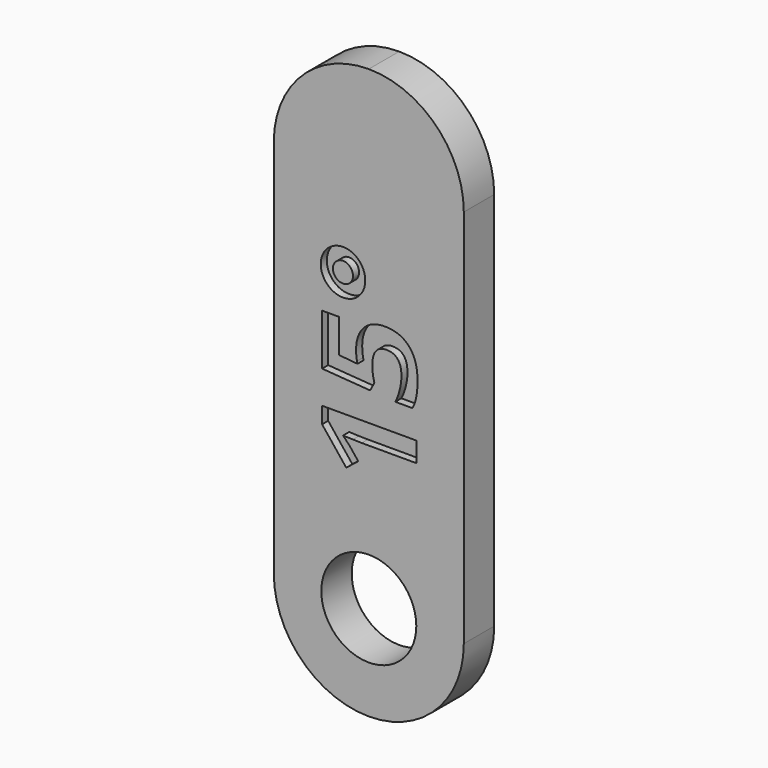
from build123d import *

# Parameters (mm, degrees)
F0_W         = 12.7
F0_H         = 38.1
F0_R         = 3.175
F1_DEPTH     = 2.54
F2_R         = 6.34999
F3_TEXT_SIZE = 8.8194444444
F4_DEPTH     = 0.508


# Not quite as in the source:
# - a fillet or chamfer is up to 0.001 mm smaller than in the source, because OpenCascade refuses the exact size
# - Text() gives the source's letters only with a copy of the font that has no kerning and outlines rounded to 1/6400 em; it was checked with that copy


with BuildPart() as f1:
    # F0 (on Front) → F1 (new body)
    with BuildSketch(Plane.XZ):
        with Locations((6.35, 19.05)):
            Rectangle(F0_W, F0_H)
        with Locations((6.35, 6.35)):
            Circle(F0_R, mode=Mode.SUBTRACT)
    extrude(amount=F1_DEPTH)

    # F2 (radius 6.35 in the source; OpenCascade refuses exactly that, so slightly less here)
    f2_edges = [f1.edges().sort_by_distance(p)[0] for p in [
        (12.7, -1.27, 0),
        (0, -1.27, 0),
        (12.7, -1.27, 38.1),
        (0, -1.27, 38.1),
    ]]
    fillet(f2_edges, radius=F2_R)

    # F3 (on face) → F4 (cut)
    with BuildSketch(Plane.XZ.offset(2.54)):
        with Locations(Location((9.525, 13.6294867622), (0, 0, 90))):
            Text('15°', F3_TEXT_SIZE, font='Open Sans', font_style=FontStyle.BOLD, text_align=(TextAlign.LEFT, TextAlign.BOTTOM))
    extrude(amount=-F4_DEPTH, mode=Mode.SUBTRACT)


solid = f1.part
